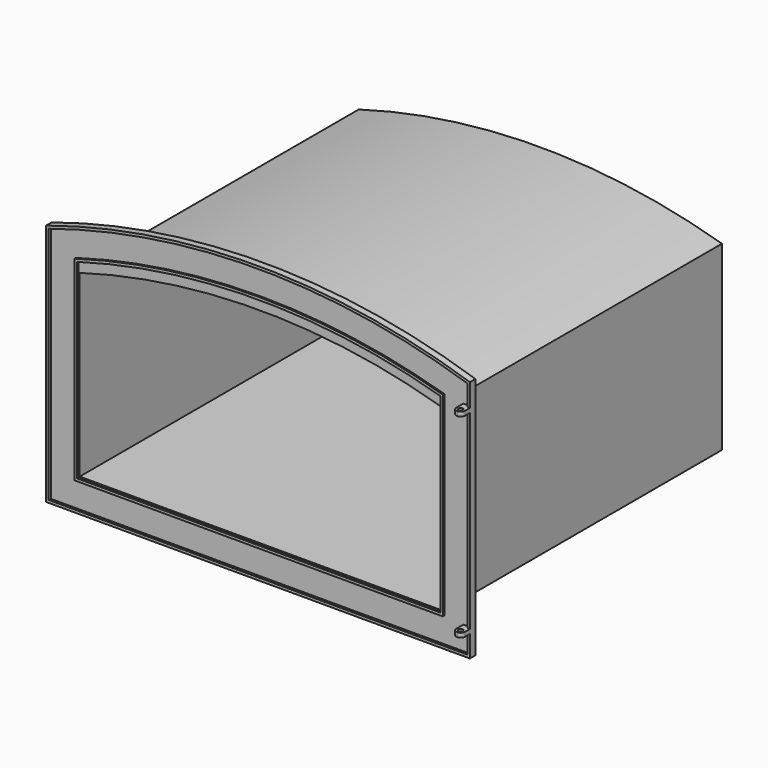
from build123d import *

# Parameters (mm, degrees)
F1_DEPTH = 405
F2_T     = -1.5
F3_DEPTH = 5
F5_DEPTH = 3
F6_DEPTH = 2
F7_W     = 10
F7_H     = 5
F8_DEPTH = 15
F9_R     = 4.99999
F11_D    = 5


# Not quite as in the source:
# - a fillet or chamfer is up to 0.001 mm smaller than in the source, because OpenCascade refuses the exact size


with BuildPart() as f1:
    # F0 (on Front) → F1 (new body)
    with BuildSketch(Plane.XZ):
        with BuildLine():
            Line((-210, -105), (210, -105))
            Line((210, -105), (210, 105))
            ThreePointArc((210, 105), (0, 135), (-210, 105))
            Line((-210, 105), (-210, -105))
        make_face()
    extrude(amount=-F1_DEPTH)

    # F2
    f2_openings = [f1.faces().sort_by_distance(p)[0] for p in [
        (0, 0, 10.213522),
    ]]
    offset(amount=F2_T, openings=f2_openings)

    # F0 (on Front) → F3 (join)
    with BuildSketch(Plane.XZ):
        with BuildLine():
            ThreePointArc((245, 141.3068160476), (0, 180), (-245, 141.3068160476))
            Line((-245, 141.3068160476), (-245, -140))
            Line((-245, -140), (245, -140))
            Line((245, -140), (245, 141.3068160476))
        make_face()
        with BuildLine():
            Line((210, 105), (210, -105))
            Line((210, -105), (-210, -105))
            Line((-210, -105), (-210, 105))
            ThreePointArc((-210, 105), (0, 135), (210, 105))
        make_face(mode=Mode.SUBTRACT)
    extrude(amount=-F3_DEPTH)

    # F4 (on face) → F5 (join)
    with BuildSketch(Plane.XZ):
        with BuildLine():
            Line((245, -140), (245, 141.3068160476))
            ThreePointArc((245, 141.3068160476), (0, 180), (-245, 141.3068160476))
            Line((-245, 141.3068160476), (-245, -140))
            Line((-245, -140), (245, -140))
        make_face()
        with BuildLine():
            Line((-242, -137), (-242, 139.1220060441))
            ThreePointArc((-242, 139.1220060441), (0, 177), (242, 139.1220060441))
            Line((242, 139.1220060441), (242, -137))
            Line((242, -137), (-242, -137))
        make_face(mode=Mode.SUBTRACT)
    extrude(amount=F5_DEPTH)

    # F4 (on face) → F6 (join)
    with BuildSketch(Plane.XZ):
        with BuildLine():
            ThreePointArc((213, 117.6663633606), (0, 148), (-213, 117.6663633606))
            Line((-213, 117.6663633606), (-213, -108))
            Line((-213, -108), (213, -108))
            Line((213, -108), (213, 117.6663633606))
        make_face()
        with BuildLine():
            ThreePointArc((-210, 115.410843293), (0, 145), (210, 115.410843293))
            Line((210, 115.410843293), (210, 105))
            Line((210, 105), (210, -105))
            Line((210, -105), (-210, -105))
            Line((-210, -105), (-210, 105))
            Line((-210, 105), (-210, 115.410843293))
        make_face(mode=Mode.SUBTRACT)
    extrude(amount=F6_DEPTH)

    # F7 (on face) → F8 (join)
    with BuildSketch(Plane.XZ):
        with Locations((240, 112.5)):
            Rectangle(F7_W, F7_H)
        with Locations((240, -112.5)):
            Rectangle(F7_W, F7_H)
    extrude(amount=F8_DEPTH)

    # F9 (radius 5 in the source; OpenCascade refuses exactly that, so slightly less here)
    f9_edges = [f1.edges().sort_by_distance(p)[0] for p in [
        (245, -15, 112.5),
        (235, -15, 112.5),
        (245, -15, -112.5),
        (235, -15, -112.5),
    ]]
    fillet(f9_edges, radius=F9_R)

    # F11 (through all)
    with Locations(Plane.XY.offset(115)):
        with Locations((240, -10)):
            Hole(F11_D / 2)


solid = f1.part
